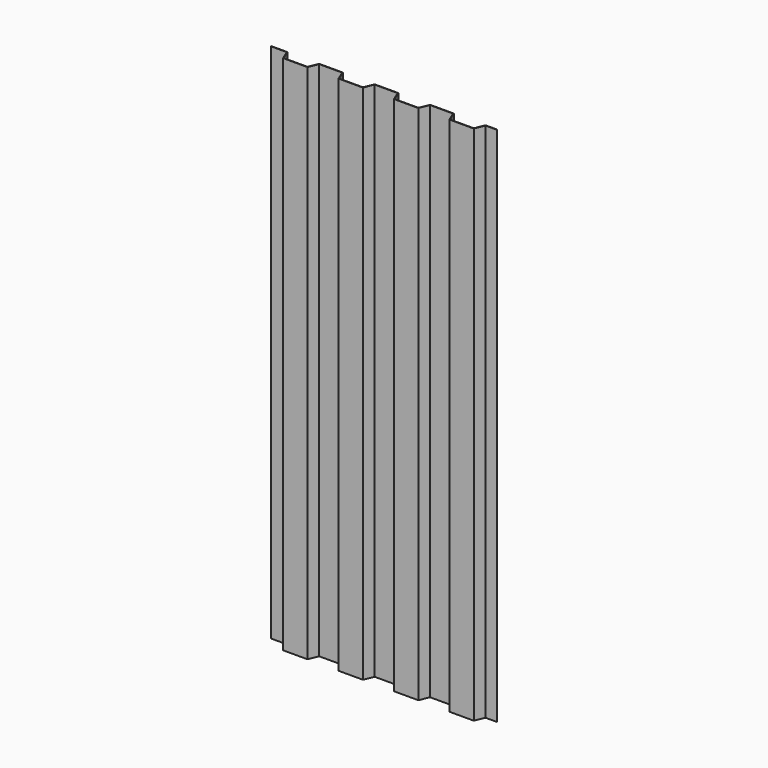
from build123d import *

# Parameters (mm, degrees)
F1_DEPTH = 2351


# Not quite as in the source:
# - ends of sketch curves that miss each other by under 0.0002 mm in the source are joined


with BuildPart() as f1:
    # F0 (on Top) → F1 (new body)
    with BuildSketch(Plane.XY):
        Polygon((0, 2), (0, 0), (72, 0), (90, -43.6), (200, -43.6), (218, 1.3e-09), (322, 1.3e-09), (340.0000000005, -43.5999999998), (450.0000001826, -43.6000004409), (468.0000001826, -4.409e-07), (572.0000001826, -4.409e-07), (590.0000001826, -43.6000004409), (700.0000001827, -43.6000004411), (718.0000001827, -4.408e-07), (822.0000003647, 0), (840.0000003647, -43.6), (950.0000003647, -43.6000000002), (968.0000003647, 0), (1019, 0), (1019, 2), (966.6619507468, 2.0000000002), (948.6619507468, -41.6), (841.3380499816, -41.6), (823.3380499816, 2), (716.6619507468, 2), (698.6619505647, -41.6000004409), (591.3380497995, -41.6000004409), (573.3380497995, 1.9999995591), (466.6619505647, 1.9999995591), (448.6619505647, -41.6000004409), (341.3380497995, -41.6000004409), (323.3380496174, 2.0000000002), (216.6619503826, 2.0000000002), (198.6619503831, -41.6), (91.3380496174, -41.6), (73.3380496174, 2), align=None)
    extrude(amount=F1_DEPTH)


solid = f1.part
